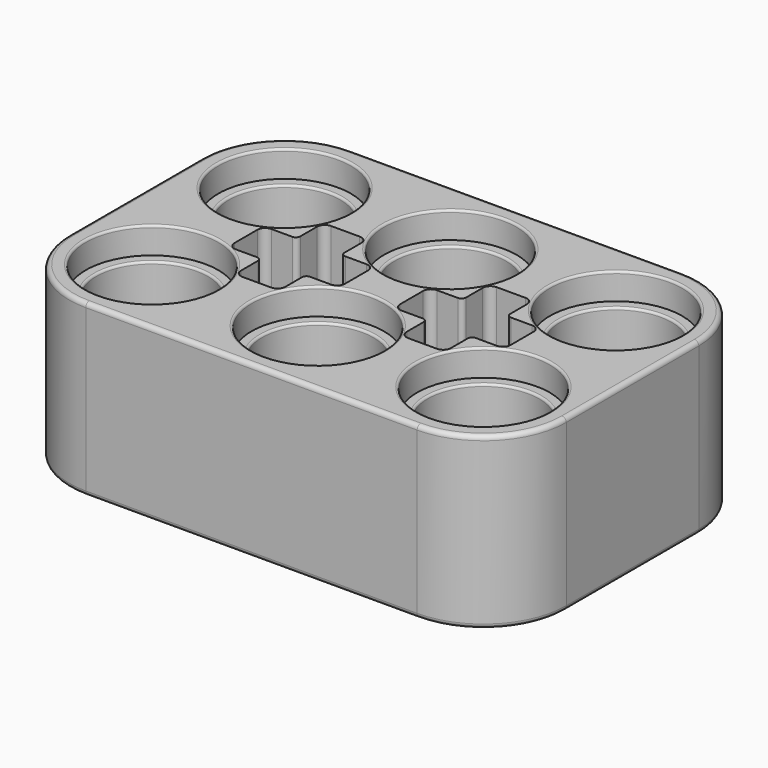
from build123d import *

# Parameters (mm, degrees)
F0_R     = 2.525
F1_DEPTH = 3.85
F2_R     = 0.2
F3_R     = 3
F4_DEPTH = 1.2
F5_R     = 0.1
F6_W     = 5
F6_H     = 0.6
F7_DEPTH = 3.85


# Not quite as in the source:
# - a feature names something its author has since deleted; it is built from what else it names


with BuildPart() as f1:
    # F0 (on Top) → F1 (new body)
    with BuildSketch(Plane.XY):
        with BuildLine():
            Line((-7.5, -7.5), (7.5, -7.5))
            ThreePointArc((7.5, -7.5), (10.1516504294, -6.4016504294), (11.25, -3.75))
            Line((11.25, -3.75), (11.25, 3.75))
            ThreePointArc((11.25, 3.75), (10.1516504294, 6.4016504294), (7.5, 7.5))
            Line((7.5, 7.5), (-7.5, 7.5))
            ThreePointArc((-7.5, 7.5), (-10.1516504294, 6.4016504294), (-11.25, 3.75))
            Line((-11.25, 3.75), (-11.25, -3.75))
            ThreePointArc((-11.25, -3.75), (-10.1516504294, -6.4016504294), (-7.5, -7.5))
        make_face()
        with Locations((-7.5, -3.75)):
            Circle(F0_R, mode=Mode.SUBTRACT)
        with Locations((0, -3.75)):
            Circle(F0_R, mode=Mode.SUBTRACT)
        with Locations((7.5, -3.75)):
            Circle(F0_R, mode=Mode.SUBTRACT)
        with Locations((-7.5, 3.75)):
            Circle(F0_R, mode=Mode.SUBTRACT)
        with Locations((0, 3.75)):
            Circle(F0_R, mode=Mode.SUBTRACT)
        with Locations((7.5, 3.75)):
            Circle(F0_R, mode=Mode.SUBTRACT)
    extrude(amount=F1_DEPTH)

    # F2
    f2_edges = [f1.edges().sort_by_distance(p)[0] for p in [
        (-10.15165, -6.40165, 3.85),
        (0, -7.5, 3.85),
        (10.15165, -6.40165, 3.85),
        (11.25, 0, 3.85),
        (10.15165, 6.40165, 3.85),
        (0, 7.5, 3.85),
        (-10.15165, 6.40165, 3.85),
        (-11.25, 0, 3.85),
        (-10.025, -3.75, 3.85),
        (-2.525, -3.75, 3.85),
        (4.975, -3.75, 3.85),
        (-10.025, 3.75, 3.85),
        (-2.525, 3.75, 3.85),
        (4.975, 3.75, 3.85),
    ]]
    fillet(f2_edges, radius=F2_R)

    # F3 (on face) → F4 (cut)
    with BuildSketch(Plane.XY.offset(3.85)):
        with Locations((-7.5, 3.75)):
            Circle(F3_R)
        with Locations((7.5, 3.75)):
            Circle(F3_R)
        with Locations((7.5, -3.75)):
            Circle(F3_R)
        with Locations((-7.5, -3.75)):
            Circle(F3_R)
        with Locations((0, 3.75)):
            Circle(F3_R)
        with Locations((0, -3.75)):
            Circle(F3_R)
    extrude(amount=-F4_DEPTH, mode=Mode.SUBTRACT)

    # F5
    f5_edges = [f1.edges().sort_by_distance(p)[0] for p in [
        (-10.5, -3.75, 3.85),
        (-10.025, -3.75, 2.65),
        (-10.5, 3.75, 3.85),
        (-10.025, 3.75, 2.65),
        (4.5, 3.75, 3.85),
        (4.975, 3.75, 2.65),
        (4.975, -3.75, 2.65),
        (4.5, -3.75, 3.85),
        (-3, 3.75, 3.85),
        (-2.525, 3.75, 2.65),
        (-3, -3.75, 3.85),
        (-2.525, -3.75, 2.65),
    ]]
    fillet(f5_edges, radius=F5_R)

    # F6 (on face) → F7 (cut, through all)
    with BuildSketch(Plane.XY.offset(3.85)):
        with BuildLine():
            ThreePointArc((-4.75, 1.2), (-4.8085786438, 1.0585786438), (-4.95, 1))
            Line((-4.95, 1), (-5.9, 1))
            ThreePointArc((-5.9, 1), (-6.1474873734, 0.8974873734), (-6.25, 0.65))
            Line((-6.25, 0.65), (-6.25, 0.3000084442))
            Line((-6.25, 0.3000084442), (-1.25, 0.3000084442))
            Line((-1.25, 0.3000084442), (-1.25, 0.65))
            ThreePointArc((-1.25, 0.65), (-1.3525126266, 0.8974873734), (-1.6, 1))
            Line((-1.6, 1), (-2.55, 1))
            ThreePointArc((-2.55, 1), (-2.6914213562, 1.0585786438), (-2.75, 1.2))
            Line((-2.75, 1.2), (-2.75, 2.15))
            ThreePointArc((-2.75, 2.15), (-2.8525126266, 2.3974873734), (-3.1, 2.5))
            Line((-3.1, 2.5), (-4.4, 2.5))
            ThreePointArc((-4.4, 2.5), (-4.6474873734, 2.3974873734), (-4.75, 2.15))
            Line((-4.75, 2.15), (-4.75, 1.2))
        make_face()
        with BuildLine():
            Line((-1.25, -0.2999915558), (-6.25, -0.2999915558))
            Line((-6.25, -0.2999915558), (-6.25, -0.65))
            ThreePointArc((-6.25, -0.65), (-6.1474873734, -0.8974873734), (-5.9, -1))
            Line((-5.9, -1), (-4.95, -1))
            ThreePointArc((-4.95, -1), (-4.8085786438, -1.0585786438), (-4.75, -1.2))
            Line((-4.75, -1.2), (-4.75, -2.15))
            ThreePointArc((-4.75, -2.15), (-4.6474873734, -2.3974873734), (-4.4, -2.5))
            Line((-4.4, -2.5), (-3.1, -2.5))
            ThreePointArc((-3.1, -2.5), (-2.8525126266, -2.3974873734), (-2.75, -2.15))
            Line((-2.75, -2.15), (-2.75, -1.2))
            ThreePointArc((-2.75, -1.2), (-2.6914213562, -1.0585786438), (-2.55, -1))
            Line((-2.55, -1), (-1.6, -1))
            ThreePointArc((-1.6, -1), (-1.3525126266, -0.8974873734), (-1.25, -0.65))
            Line((-1.25, -0.65), (-1.25, -0.2999915558))
        make_face()
        with Locations((-3.75, 8.4442e-06)):
            Rectangle(F6_W, F6_H)
        with BuildLine():
            Line((5.9, 1), (4.95, 1))
            ThreePointArc((4.95, 1), (4.8085786438, 1.0585786438), (4.75, 1.2))
            Line((4.75, 1.2), (4.75, 2.15))
            ThreePointArc((4.75, 2.15), (4.6474873734, 2.3974873734), (4.4, 2.5))
            Line((4.4, 2.5), (3.1, 2.5))
            ThreePointArc((3.1, 2.5), (2.8525126266, 2.3974873734), (2.75, 2.15))
            Line((2.75, 2.15), (2.75, 1.2))
            ThreePointArc((2.75, 1.2), (2.6914213562, 1.0585786438), (2.55, 1))
            Line((2.55, 1), (1.6, 1))
            ThreePointArc((1.6, 1), (1.3525126266, 0.8974873734), (1.25, 0.65))
            Line((1.25, 0.65), (1.25, 0.3000084442))
            Line((1.25, 0.3000084442), (6.25, 0.3000084442))
            Line((6.25, 0.3000084442), (6.25, 0.65))
            ThreePointArc((6.25, 0.65), (6.1474873734, 0.8974873734), (5.9, 1))
        make_face()
        with Locations((3.75, 8.4442e-06)):
            Rectangle(F6_W, F6_H)
        with BuildLine():
            Line((6.25, -0.65), (6.25, -0.2999915558))
            Line((6.25, -0.2999915558), (1.25, -0.2999915558))
            Line((1.25, -0.2999915558), (1.25, -0.65))
            ThreePointArc((1.25, -0.65), (1.3525126266, -0.8974873734), (1.6, -1))
            Line((1.6, -1), (2.55, -1))
            ThreePointArc((2.55, -1), (2.6914213562, -1.0585786438), (2.75, -1.2))
            Line((2.75, -1.2), (2.75, -2.15))
            ThreePointArc((2.75, -2.15), (2.8525126266, -2.3974873734), (3.1, -2.5))
            Line((3.1, -2.5), (4.4, -2.5))
            ThreePointArc((4.4, -2.5), (4.6474873734, -2.3974873734), (4.75, -2.15))
            Line((4.75, -2.15), (4.75, -1.2))
            ThreePointArc((4.75, -1.2), (4.8085786438, -1.0585786438), (4.95, -1))
            Line((4.95, -1), (5.9, -1))
            ThreePointArc((5.9, -1), (6.1474873734, -0.8974873734), (6.25, -0.65))
        make_face()
    extrude(amount=-F7_DEPTH, mode=Mode.SUBTRACT)

    # F8: F1 across plane


with BuildPart() as f1_1:
    add(f1.part)
    add(f1.part.mirror(Plane.XY))


solid = f1_1.part
